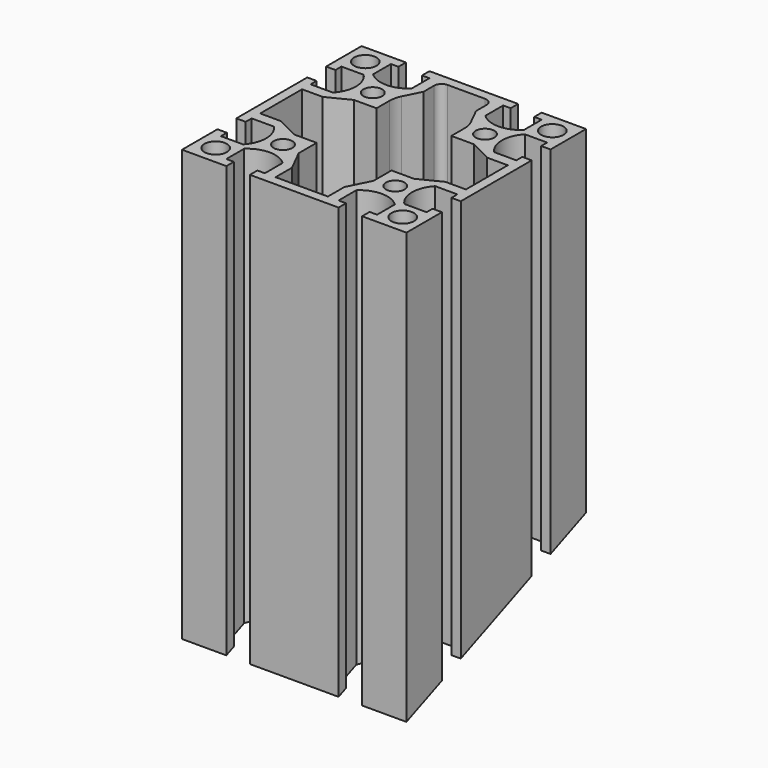
from build123d import *

# Parameters (mm, degrees)
F0_R          = 3
F0_R_2        = 2.5
F1_DEPTH      = 140
F2_R          = 2
F3_R          = 7
F6_DEPTH      = 30
F6_DEPTH_BACK = 30
F7_W          = 131.1645284295
F7_H          = 50.7057756186
F8_DEPTH      = 30
F8_DEPTH_BACK = 30


# Not quite as in the source:
# - a feature names something its author has since deleted; it is built from what else it names


with BuildPart() as f1:
    # F0 (on Top) → F1 (new body)
    with BuildSketch(Plane.XY):
        with BuildLine():
            Line((18.15, -30), (30, -30))
            Line((30, -30), (30, -18.15))
            Line((30, -18.15), (27.5, -18.15))
            Line((27.5, -18.15), (27.5, -20.15))
            Line((27.5, -20.15), (21.5477069044, -20.15))
            ThreePointArc((21.5477069044, -20.15), (19.5, -15), (21.5477069044, -9.85))
            Line((21.5477069044, -9.85), (27.5, -9.85))
            Line((27.5, -9.85), (27.5, -11.85))
            Line((27.5, -11.85), (30, -11.85))
            Line((30, -11.85), (30, 11.85))
            Line((30, 11.85), (27.5, 11.85))
            Line((27.5, 11.85), (27.5, 9.85))
            Line((27.5, 9.85), (21.5477069044, 9.85))
            ThreePointArc((21.5477069044, 9.85), (19.5, 15), (21.5477069044, 20.15))
            Line((21.5477069044, 20.15), (27.5, 20.15))
            Line((27.5, 20.15), (27.5, 18.15))
            Line((27.5, 18.15), (30, 18.15))
            Line((30, 18.15), (30, 30))
            Line((30, 30), (18.15, 30))
            Line((18.15, 30), (18.15, 27.5))
            Line((18.15, 27.5), (20.15, 27.5))
            Line((20.15, 27.5), (20.15, 21.5477069044))
            ThreePointArc((20.15, 21.5477069044), (15, 19.5), (9.85, 21.5477069044))
            Line((9.85, 21.5477069044), (9.85, 27.5))
            Line((9.85, 27.5), (11.85, 27.5))
            Line((11.85, 27.5), (11.85, 30))
            Line((11.85, 30), (-11.85, 30))
            Line((-11.85, 30), (-11.85, 27.5))
            Line((-11.85, 27.5), (-9.85, 27.5))
            Line((-9.85, 27.5), (-9.85, 21.5477069044))
            ThreePointArc((-9.85, 21.5477069044), (-15, 19.5), (-20.15, 21.5477069044))
            Line((-20.15, 21.5477069044), (-20.15, 27.5))
            Line((-20.15, 27.5), (-18.15, 27.5))
            Line((-18.15, 27.5), (-18.15, 30))
            Line((-18.15, 30), (-30, 30))
            Line((-30, 30), (-30, 18.15))
            Line((-30, 18.15), (-27.5, 18.15))
            Line((-27.5, 18.15), (-27.5, 20.15))
            Line((-27.5, 20.15), (-21.5477069044, 20.15))
            ThreePointArc((-21.5477069044, 20.15), (-19.5, 15), (-21.5477069044, 9.85))
            Line((-21.5477069044, 9.85), (-27.5, 9.85))
            Line((-27.5, 9.85), (-27.5, 11.85))
            Line((-27.5, 11.85), (-30, 11.85))
            Line((-30, 11.85), (-30, -11.85))
            Line((-30, -11.85), (-27.5, -11.85))
            Line((-27.5, -11.85), (-27.5, -9.85))
            Line((-27.5, -9.85), (-21.5477069044, -9.85))
            ThreePointArc((-21.5477069044, -9.85), (-19.5, -15), (-21.5477069044, -20.15))
            Line((-21.5477069044, -20.15), (-27.5, -20.15))
            Line((-27.5, -20.15), (-27.5, -18.15))
            Line((-27.5, -18.15), (-30, -18.15))
            Line((-30, -18.15), (-30, -30))
            Line((-30, -30), (-18.15, -30))
            Line((-18.15, -30), (-18.15, -27.5))
            Line((-18.15, -27.5), (-20.15, -27.5))
            Line((-20.15, -27.5), (-20.15, -21.5477069044))
            ThreePointArc((-20.15, -21.5477069044), (-15, -19.5), (-9.85, -21.5477069044))
            Line((-9.85, -21.5477069044), (-9.85, -27.5))
            Line((-9.85, -27.5), (-11.85, -27.5))
            Line((-11.85, -27.5), (-11.85, -30))
            Line((-11.85, -30), (11.85, -30))
            Line((11.85, -30), (11.85, -27.5))
            Line((11.85, -27.5), (9.85, -27.5))
            Line((9.85, -27.5), (9.85, -21.5477069044))
            ThreePointArc((9.85, -21.5477069044), (15, -19.5), (20.15, -21.5477069044))
            Line((20.15, -21.5477069044), (20.15, -27.5))
            Line((20.15, -27.5), (18.15, -27.5))
            Line((18.15, -27.5), (18.15, -30))
        make_face()
        with Locations((-25, -25)):
            Circle(F0_R, mode=Mode.SUBTRACT)
        with Locations((-15, -15)):
            Circle(F0_R_2, mode=Mode.SUBTRACT)
        with Locations((25, -25)):
            Circle(F0_R, mode=Mode.SUBTRACT)
        with Locations((15, -15)):
            Circle(F0_R_2, mode=Mode.SUBTRACT)
        with Locations((-25, 25)):
            Circle(F0_R, mode=Mode.SUBTRACT)
        with Locations((-15, 15)):
            Circle(F0_R_2, mode=Mode.SUBTRACT)
        Polygon((-7, 22), (-7, 27.5), (0, 27.5), (7, 27.5), (7, 22), (10, 16), (10, 10), (16, 10), (22, 7), (27.5, 7), (27.5, 0), (27.5, -7), (22, -7), (16, -10), (10, -10), (10, -16), (7, -22), (7, -27.5), (0, -27.5), (-7, -27.5), (-7, -22), (-10, -16), (-10, -10), (-16, -10), (-22, -7), (-27.5, -7), (-27.5, 0), (-27.5, 7), (-22, 7), (-16, 10), (-10, 10), (-10, 16), align=None, mode=Mode.SUBTRACT)
        with Locations((15, 15)):
            Circle(F0_R_2, mode=Mode.SUBTRACT)
        with Locations((25, 25)):
            Circle(F0_R, mode=Mode.SUBTRACT)
    extrude(amount=F1_DEPTH)

    # F2
    f2_edges = [f1.edges().sort_by_distance(p)[0] for p in [
        (-7, 27.5, 70),
        (7, 27.5, 70),
    ]]
    fillet(f2_edges, radius=F2_R)

    # F3
    f3_edges = [f1.edges().sort_by_distance(p)[0] for p in [
        (-10, 16, 70),
        (10, 16, 70),
    ]]
    fillet(f3_edges, radius=F3_R)

    # F5 (on Right) → F6 (cut, two sides)
    with BuildSketch(Plane.YZ) as f6_sk:
        Polygon((214.5999793503, -135.2321386172), (130.9673605882, 66.674863855), (-30, 0), (53.6326187621, -201.9070024722), align=None)
        Polygon((30, 140), (-2.0081647111, 217.2745453523), (-162.3392477394, 150.863236292), (-130.3310830283, 73.5886909397), align=None)
    extrude(amount=-F6_DEPTH, mode=Mode.SUBTRACT)
    extrude(f6_sk.sketch, amount=F6_DEPTH_BACK, mode=Mode.SUBTRACT)

    # F7 (on Right) → F8 (cut, two sides)
    with BuildSketch(Plane.YZ) as f8_sk:
        with Locations((35.5822642148, 140.5000740669)):
            Rectangle(F7_W, F7_H)
    extrude(amount=F8_DEPTH, mode=Mode.SUBTRACT)
    extrude(f8_sk.sketch, amount=-F8_DEPTH_BACK, mode=Mode.SUBTRACT)


solid = f1.part
